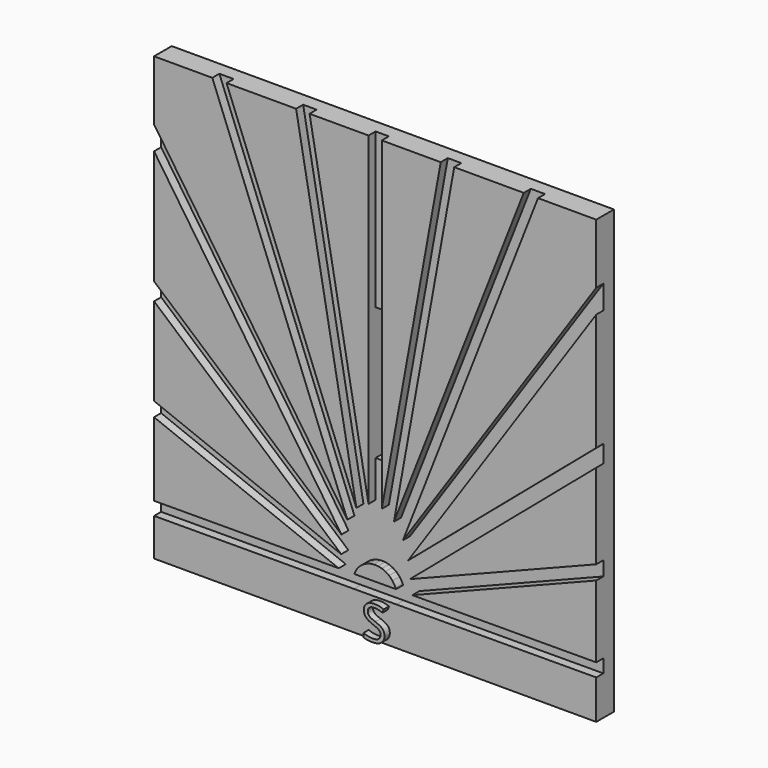
from build123d import *

# Parameters (mm, degrees)
F0_W          = 100
F0_H          = 100
F0_W_2        = 3
F0_H_2        = 30
F1_DEPTH      = 5
F3_DEPTH      = 2
F5_DEPTH      = 2
F7_DEPTH      = 2
F9_DEPTH      = 2
F11_DEPTH     = 2
F12_W         = 1.5
F12_H         = 35
F13_DEPTH     = 2
F15_DEPTH     = 2
F17_DEPTH     = 2
F19_DEPTH     = 2
F21_DEPTH     = 2
F23_DEPTH     = 2
F25_DEPTH     = 2
F26_TEXT_SIZE = 10.6048053024
F27_DEPTH     = 1.5


# Not quite as in the source:
# - a feature names something its author has since deleted; it is built from what else it names
# - Text() gives the source's letters only with a copy of the font that has no kerning and outlines rounded to 1/6400 em; it was checked with that copy


with BuildPart() as f1:
    # F0 (on Front) → F1 (new body)
    with BuildSketch(Plane.XZ):
        Rectangle(F0_W, F0_H)
        Rectangle(F0_W_2, F0_H_2, mode=Mode.SUBTRACT)
    extrude(amount=F1_DEPTH)

    # F2 (on face) → F3 (cut)
    with BuildSketch(Plane.XZ.offset(5)):
        with BuildLine():
            Line((-50, -20.2338771656), (-4.64984554, -38.1618116379))
            ThreePointArc((-4.64984554, -38.1618116379), (-4.3170305173, -37.4774521784), (-3.8842134325, -36.8515263998))
            Line((-3.8842134325, -36.8515263998), (-50, -18.6209203619))
            Line((-50, -18.6209203619), (-50, -20.2338771656))
        make_face()
        with BuildLine():
            ThreePointArc((-4.9871264497, -39.6414337238), (-4.8749489907, -38.8887519007), (-4.64984554, -38.1618116379))
            Line((-4.64984554, -38.1618116379), (-50, -20.2338771656))
            Line((-50, -20.2338771656), (-50, -21.8468339693))
            Line((-50, -21.8468339693), (-4.9871264497, -39.6414337238))
        make_face()
    extrude(amount=-F3_DEPTH, mode=Mode.SUBTRACT)

    # F4 (on face) → F5 (cut)
    with BuildSketch(Plane.XZ.offset(5)):
        with BuildLine():
            ThreePointArc((-3.7832139188, -36.7308575368), (-3.243278159, -36.1945898009), (-2.6282133255, -35.7464726737))
            Line((-2.6282133255, -35.7464726737), (-50, 5.1883310939))
            Line((-50, 5.1883310939), (-50, 3.2058896668))
            Line((-50, 3.2058896668), (-3.7832139188, -36.7308575368))
        make_face()
        with BuildLine():
            ThreePointArc((-3.8842134325, -36.8515263998), (-3.8341884135, -36.790794614), (-3.7832139188, -36.7308575368))
            Line((-3.7832139188, -36.7308575368), (-50, 3.2058896668))
            Line((-50, 3.2058896668), (-50, 1.2234482398))
            Line((-50, 1.2234482398), (-7.6694411179, -35.3551408921))
            Line((-7.6694411179, -35.3551408921), (-3.8842134325, -36.8515263998))
        make_face()
    extrude(amount=-F5_DEPTH, mode=Mode.SUBTRACT)

    # F6 (on face) → F7 (cut)
    with BuildSketch(Plane.XZ.offset(5)):
        with BuildLine():
            ThreePointArc((-2.6282133255, -35.7464726737), (-2.0489749507, -35.4391117476), (-1.4344952039, -35.2101958798))
            Line((-1.4344952039, -35.2101958798), (-50, 36.4399153359))
            Line((-50, 36.4399153359), (-50, 33.7664639919))
            Line((-50, 33.7664639919), (-3.2434623217, -35.2148250688))
            Line((-3.2434623217, -35.2148250688), (-2.6282133255, -35.7464726737))
        make_face()
        Polygon((-7.617482449, -31.4351564483), (-3.2434623217, -35.2148250688), (-50, 33.7664639919), (-50, 31.0930126479), align=None)
    extrude(amount=-F7_DEPTH, mode=Mode.SUBTRACT)

    # F8 (on face) → F9 (cut)
    with BuildSketch(Plane.XZ.offset(5)):
        Polygon((-2.474712004, -33.6755335773), (-35.2162641832, 50), (-36.8270080816, 50), (-6.2851780983, -28.0538413785), align=None)
        with BuildLine():
            Line((-33.6055202847, 50), (-35.2162641832, 50))
            Line((-35.2162641832, 50), (-2.474712004, -33.6755335773))
            Line((-2.474712004, -33.6755335773), (-1.4344952039, -35.2101958798))
            ThreePointArc((-1.4344952039, -35.2101958798), (-0.8933582622, -35.0804562188), (-0.3411557717, -35.0116523037))
            Line((-0.3411557717, -35.0116523037), (-33.6055202847, 50))
        make_face()
    extrude(amount=-F9_DEPTH, mode=Mode.SUBTRACT)

    # F10 (on face) → F11 (cut)
    with BuildSketch(Plane.XZ.offset(5)):
        Polygon((-4.2435033714, -25.0386670334), (-1.396833111, -32.313723868), (-16.3557720059, 50), (-17.8803403672, 50), align=None)
        with BuildLine():
            ThreePointArc((-0.3411557717, -35.0116523037), (0.1415799083, -35.002004889), (0.6229953454, -35.0389641405))
            Line((0.6229953454, -35.0389641405), (-14.8312036446, 50))
            Line((-14.8312036446, 50), (-16.3557720059, 50))
            Line((-16.3557720059, 50), (-1.396833111, -32.313723868))
            Line((-1.396833111, -32.313723868), (-0.3411557717, -35.0116523037))
        make_face()
    extrude(amount=-F11_DEPTH, mode=Mode.SUBTRACT)

    # F12 (on face) → F13 (cut)
    with BuildSketch(Plane.XZ.offset(5)):
        with Locations((-0.75, 32.5)):
            Rectangle(F12_W, F12_H)
        with Locations((0.75, 32.5)):
            Rectangle(F12_W, F12_H)
        Polygon((0, -31.6108421866), (0, -15), (-1.5, -15), (-1.5, -23.3568753331), align=None)
        with BuildLine():
            Line((1.5, -15), (0, -15))
            Line((0, -15), (0, -31.6108421866))
            Line((0, -31.6108421866), (0.6229953454, -35.0389641405))
            ThreePointArc((0.6229953454, -35.0389641405), (1.0658001895, -35.114913516), (1.5, -35.2303039929))
            Line((1.5, -35.2303039929), (1.5, -15))
        make_face()
        with BuildLine():
            Line((0, -35), (0, -31.6108421866))
            Line((0, -31.6108421866), (-1.5, -23.3568753331))
            Line((-1.5, -23.3568753331), (-1.5, -35.2303039929))
            ThreePointArc((-1.5, -35.2303039929), (-0.7587884964, -35.0579113709), (0, -35))
        make_face()
    extrude(amount=-F13_DEPTH, mode=Mode.SUBTRACT)

    # F14 (on face) → F15 (cut)
    with BuildSketch(Plane.XZ.offset(5)):
        with BuildLine():
            ThreePointArc((1.5, -35.2303039929), (1.9220891442, -35.3842039341), (2.3286597684, -35.5753707858))
            Line((2.3286597684, -35.5753707858), (17.8803403672, 50))
            Line((17.8803403672, 50), (16.3557720059, 50))
            Line((16.3557720059, 50), (1.5, -31.7460331465))
            Line((1.5, -31.7460331465), (1.5, -35.2303039929))
        make_face()
        Polygon((1.5, -23.3568753331), (1.5, -31.7460331465), (16.3557720059, 50), (14.8312036446, 50), align=None)
    extrude(amount=-F15_DEPTH, mode=Mode.SUBTRACT)

    # F16 (on face) → F17 (cut)
    with BuildSketch(Plane.XZ.offset(5)):
        Polygon((4.2435033714, -25.0386670334), (2.8466702604, -32.7249431654), (35.2162641832, 50), (33.6055202847, 50), align=None)
        with BuildLine():
            ThreePointArc((2.3286597684, -35.5753707858), (2.7445745541, -35.8206088342), (3.1348959835, -36.1048200076))
            Line((3.1348959835, -36.1048200076), (36.8270080816, 50))
            Line((36.8270080816, 50), (35.2162641832, 50))
            Line((35.2162641832, 50), (2.8466702604, -32.7249431654))
            Line((2.8466702604, -32.7249431654), (2.3286597684, -35.5753707858))
        make_face()
    extrude(amount=-F17_DEPTH, mode=Mode.SUBTRACT)

    # F18 (on face) → F19 (cut)
    with BuildSketch(Plane.XZ.offset(5)):
        Polygon((3.8104660943, -34.3783078012), (50, 33.7664639919), (50, 36.4399153359), (6.2851780983, -28.0538413785), align=None)
        with BuildLine():
            Line((50, 31.0930126479), (50, 33.7664639919))
            Line((50, 33.7664639919), (3.8104660943, -34.3783078012))
            Line((3.8104660943, -34.3783078012), (3.1348959835, -36.1048200076))
            ThreePointArc((3.1348959835, -36.1048200076), (3.5483211746, -36.4772997798), (3.9177952177, -36.893413347))
            Line((3.9177952177, -36.893413347), (50, 31.0930126479))
        make_face()
    extrude(amount=-F19_DEPTH, mode=Mode.SUBTRACT)

    # F20 (on face) → F21 (cut)
    with BuildSketch(Plane.XZ.offset(5)):
        Polygon((4.2867094758, -36.3491433403), (50, 2.5834393534), (50, 4.5537221697), (7.4459328661, -31.688248571), align=None)
        with BuildLine():
            Line((50, 0.613156537), (50, 2.5834393534))
            Line((50, 2.5834393534), (4.2867094758, -36.3491433403))
            Line((4.2867094758, -36.3491433403), (3.9177952177, -36.893413347))
            ThreePointArc((3.9177952177, -36.893413347), (4.2998227644, -37.4482311635), (4.6038054569, -38.049365407))
            Line((4.6038054569, -38.049365407), (50, 0.613156537))
        make_face()
    extrude(amount=-F21_DEPTH, mode=Mode.SUBTRACT)

    # F22 (on face) → F23 (cut)
    with BuildSketch(Plane.XZ.offset(5)):
        with BuildLine():
            Line((50, -21.8468339693), (50, -20.2338771656))
            Line((50, -20.2338771656), (4.64984554, -38.1618116379))
            ThreePointArc((4.64984554, -38.1618116379), (4.8749489907, -38.8887519007), (4.9871264497, -39.6414337238))
            Line((4.9871264497, -39.6414337238), (50, -21.8468339693))
        make_face()
        with BuildLine():
            Line((4.64984554, -38.1618116379), (50, -20.2338771656))
            Line((50, -20.2338771656), (50, -18.6209203619))
            Line((50, -18.6209203619), (7.8520180432, -35.2829641335))
            Line((7.8520180432, -35.2829641335), (4.6038054569, -38.049365407))
            ThreePointArc((4.6038054569, -38.049365407), (4.6271670849, -38.105448663), (4.64984554, -38.1618116379))
        make_face()
    extrude(amount=-F23_DEPTH, mode=Mode.SUBTRACT)

    # F24 (on face) → F25 (cut)
    with BuildSketch(Plane.XZ.offset(5)):
        with BuildLine():
            Line((-50, -40), (-4.9973954823, -39.8386358368))
            ThreePointArc((-4.9973954823, -39.8386358368), (-4.9932345951, -39.7399840799), (-4.9871264497, -39.6414337238))
            Line((-4.9871264497, -39.6414337238), (-8.2531526033, -38.3503002412))
            Line((-8.2531526033, -38.3503002412), (-50, -38.4999903573))
            Line((-50, -38.4999903573), (-50, -40))
        make_face()
        with BuildLine():
            ThreePointArc((-4.8176501943, -41.3380009735), (-4.964454085, -40.595143376), (-4.9973954823, -39.8386358368))
            Line((-4.9973954823, -39.8386358368), (-50, -40))
            Line((-50, -40), (-50, -41.5000096427))
            Line((-50, -41.5000096427), (-4.8176501943, -41.3380009735))
        make_face()
        with BuildLine():
            Line((-4.9973954823, -39.8386358368), (4.9961098011, -39.802802497))
            ThreePointArc((4.9961098011, -39.802802497), (4.992270173, -39.7220818111), (4.9871264497, -39.6414337238))
            ThreePointArc((4.9871264497, -39.6414337238), (4.8912593569, -38.9628973514), (4.7035144358, -38.3038420026))
            Line((4.7035144358, -38.3038420026), (-4.7155570362, -38.3376156165))
            ThreePointArc((-4.7155570362, -38.3376156165), (-4.8949465902, -38.9804423122), (-4.9871264497, -39.6414337238))
            ThreePointArc((-4.9871264497, -39.6414337238), (-4.9932345951, -39.7399840799), (-4.9973954823, -39.8386358368))
        make_face()
        with BuildLine():
            ThreePointArc((4.8271214322, -41.303418075), (4.956591932, -40.6574164733), (5, -40))
            ThreePointArc((5, -40), (4.9990273557, -39.9013820645), (4.9961098011, -39.802802497))
            Line((4.9961098011, -39.802802497), (-4.9973954823, -39.8386358368))
            ThreePointArc((-4.9973954823, -39.8386358368), (-4.964454085, -40.595143376), (-4.8176501943, -41.3380009735))
            Line((-4.8176501943, -41.3380009735), (4.8271214322, -41.303418075))
        make_face()
        with BuildLine():
            ThreePointArc((4.9871264497, -39.6414337238), (4.992270173, -39.7220818111), (4.9961098011, -39.802802497))
            Line((4.9961098011, -39.802802497), (50, -39.6414337238))
            Line((50, -39.6414337238), (50, -38.1414240811))
            Line((50, -38.1414240811), (8.4042388552, -38.2905724529))
            Line((8.4042388552, -38.2905724529), (4.9871264497, -39.6414337238))
        make_face()
        with BuildLine():
            ThreePointArc((4.9961098011, -39.802802497), (4.9990273557, -39.9013820645), (5, -40))
            ThreePointArc((5, -40), (4.956591932, -40.6574164733), (4.8271214322, -41.303418075))
            Line((4.8271214322, -41.303418075), (50, -41.1414433665))
            Line((50, -41.1414433665), (50, -39.6414337238))
            Line((50, -39.6414337238), (4.9961098011, -39.802802497))
        make_face()
        with BuildLine():
            Line((-8.2531526033, -38.3503002412), (-4.9871264497, -39.6414337238))
            ThreePointArc((-4.9871264497, -39.6414337238), (-4.8949465902, -38.9804423122), (-4.7155570362, -38.3376156165))
            Line((-4.7155570362, -38.3376156165), (-8.2531526033, -38.3503002412))
        make_face()
        with BuildLine():
            ThreePointArc((4.7035144358, -38.3038420026), (4.8912593569, -38.9628973514), (4.9871264497, -39.6414337238))
            Line((4.9871264497, -39.6414337238), (8.4042388552, -38.2905724529))
            Line((8.4042388552, -38.2905724529), (4.7035144358, -38.3038420026))
        make_face()
    extrude(amount=-F25_DEPTH, mode=Mode.SUBTRACT)

    # F26 (on face) → F27 (join)
    with BuildSketch(Plane.XZ.offset(5)):
        with Locations((-2, -49.5)):
            Text('S', F26_TEXT_SIZE, font='Open Sans', text_align=(TextAlign.LEFT, TextAlign.BOTTOM))
    extrude(amount=F27_DEPTH)


solid = f1.part
